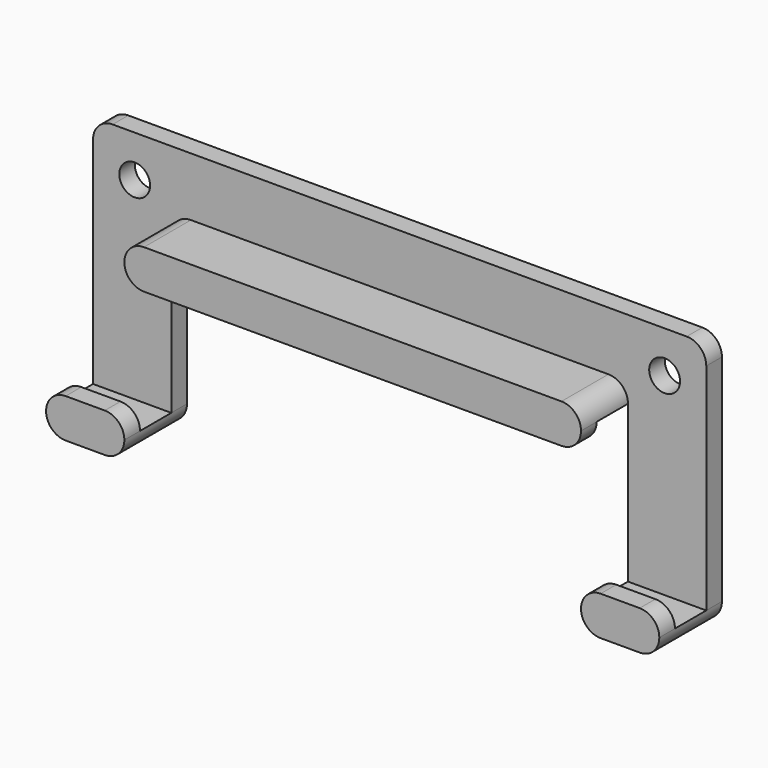
from build123d import *

# Parameters (mm, degrees)
F0_R     = 2.5019
F1_DEPTH = 3.175
F2_W     = 12.7
F2_H     = 3.175
F2_W_2   = 74.0918
F3_DEPTH = 9.525
F4_W     = 12.7
F4_H     = 3.175
F5_W     = 12.7
F5_H     = 3.175
F6_DEPTH = 3.175
F7_W     = 74.0918
F7_H     = 3.175
F8_DEPTH = 3.175
F9_R     = 3.17499


# Not quite as in the source:
# - a fillet or chamfer is up to 0.001 mm smaller than in the source, because OpenCascade refuses the exact size
# - a feature names something its author has since deleted; it is built from what else it names


with BuildPart() as f1:
    # F0 (on Front) → F1 (new body)
    with BuildSketch(Plane.XZ):
        Polygon((49.7459, 20.6375), (-49.7459, 20.6375), (-49.7459, -20.6375), (-37.0459, -20.6375), (-37.0459, 7.9375), (37.0459, 7.9375), (37.0459, -20.6375), (49.7459, -20.6375), align=None)
        with Locations((-42.9895, 13.8811)):
            Circle(F0_R, mode=Mode.SUBTRACT)
        with Locations((42.9895, 13.8811)):
            Circle(F0_R, mode=Mode.SUBTRACT)
    extrude(amount=F1_DEPTH)

    # F2 (on face) → F3 (join)
    with BuildSketch(Plane.XZ.offset(3.175)):
        with Locations((-43.3959, -19.05)):
            Rectangle(F2_W, F2_H)
        with Locations((0, 9.525)):
            Rectangle(F2_W_2, F2_H)
        with Locations((43.3959, -19.05)):
            Rectangle(F2_W, F2_H)
    extrude(amount=F3_DEPTH)

    # F4 (on face) + F5 (on face) → F6 (join)
    with BuildSketch(Plane.XY.offset(-17.4625)):
        with Locations((-43.3959, -11.1125)):
            Rectangle(F4_W, F4_H)
    with BuildSketch(Plane.XY.offset(-17.4625)):
        with Locations((43.3959, -11.1125)):
            Rectangle(F5_W, F5_H)
    extrude(amount=F6_DEPTH)

    # F7 (on face) → F8 (join)
    with BuildSketch(Plane(origin=(0, 0, 7.9375), x_dir=(1, 0, 0), z_dir=(0, 0, -1))):
        with Locations((0, 11.1125)):
            Rectangle(F7_W, F7_H)
    extrude(amount=F8_DEPTH)

    # F9 (radius 3.175 in the source; OpenCascade refuses exactly that, so slightly less here)
    f9_edges = [f1.edges().sort_by_distance(p)[0] for p in [
        (-49.7459, -1.5875, 20.6375),
        (-49.7459, -6.35, -20.6375),
        (-49.7459, -11.1125, -14.2875),
        (-37.0459, -7.9375, 11.1125),
        (-37.0459, -11.1125, 4.7625),
        (-37.0459, -11.1125, -14.2875),
        (-37.0459, -6.35, -20.6375),
        (49.7459, -1.5875, 20.6375),
        (49.7459, -6.35, -20.6375),
        (37.0459, -7.9375, 11.1125),
        (37.0459, -11.1125, 4.7625),
        (37.0459, -11.1125, -14.2875),
        (37.0459, -6.35, -20.6375),
        (49.7459, -11.1125, -14.2875),
    ]]
    fillet(f9_edges, radius=F9_R)


solid = f1.part
